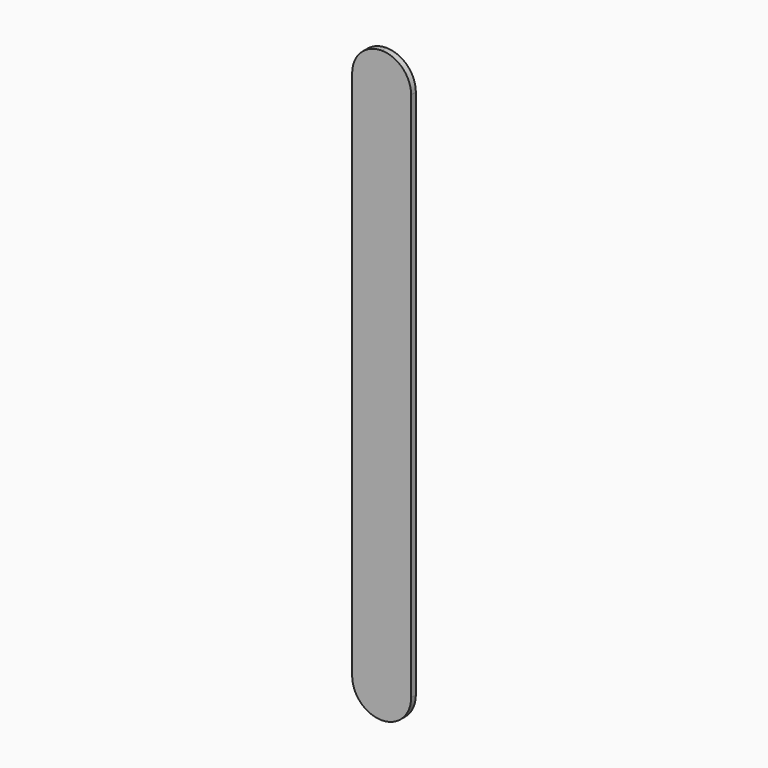
from build123d import *

# Parameters (mm, degrees)
F0_W     = 10
F0_H     = 100
F1_DEPTH = 0.5
F2_R     = 5
F3_R     = 4.99999
F4_R     = 5
F5_R     = 4.99999


# Not quite as in the source:
# - a fillet or chamfer is up to 0.001 mm smaller than in the source, because OpenCascade refuses the exact size


with BuildPart() as f1:
    # F0 (on Front) → F1 (new body, symmetric)
    with BuildSketch(Plane.XZ):
        with Locations((5, 50)):
            Rectangle(F0_W, F0_H)
    extrude(amount=F1_DEPTH, both=True)

    # F2
    f2_edges = [f1.edges().sort_by_distance(p)[0] for p in [
        (0, 0, 100),
    ]]
    fillet(f2_edges, radius=F2_R)

    # F3 (radius 5 in the source; OpenCascade refuses exactly that, so slightly less here)
    f3_edges = [f1.edges().sort_by_distance(p)[0] for p in [
        (10, 0, 100),
    ]]
    fillet(f3_edges, radius=F3_R)

    # F4
    f4_edges = [f1.edges().sort_by_distance(p)[0] for p in [
        (0, 0, 0),
    ]]
    fillet(f4_edges, radius=F4_R)

    # F5 (radius 5 in the source; OpenCascade refuses exactly that, so slightly less here)
    f5_edges = [f1.edges().sort_by_distance(p)[0] for p in [
        (10, 0, 0),
    ]]
    fillet(f5_edges, radius=F5_R)


solid = f1.part
